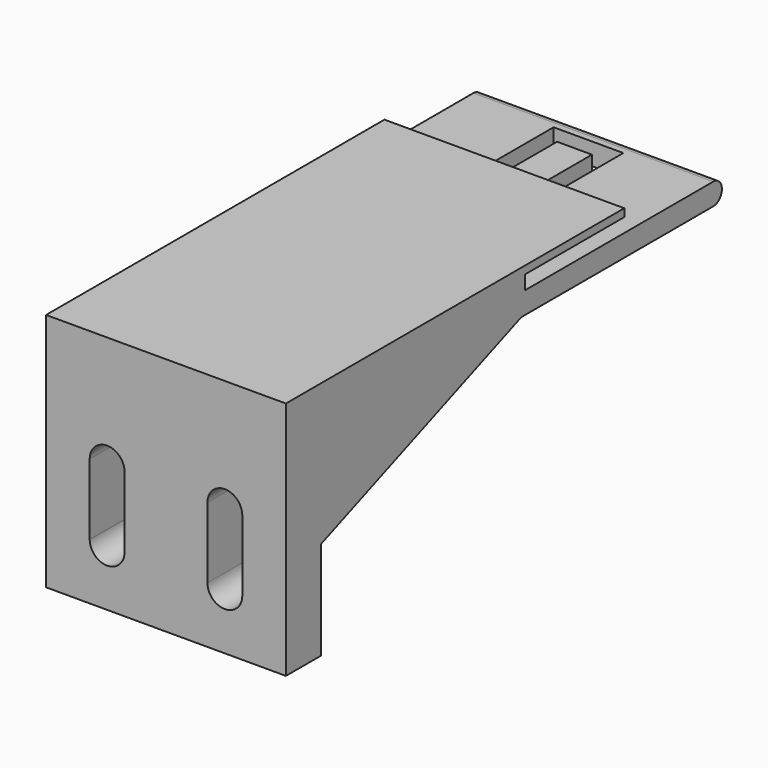
from build123d import *

# Parameters (mm, degrees)
F0_W      = 17.4625
F0_H      = 34.925
F1_DEPTH  = 6.35
F2_W      = 34.925
F2_H      = 6.35
F3_DEPTH  = 73.025
F5_DEPTH  = 3.175
F7_DEPTH  = 3.175
F8_W      = 34.925
F8_H      = 3.175
F9_DEPTH  = 17.78
F10_W     = 34.925
F10_H     = 1.143
F10_H_2   = 0.889
F11_DEPTH = 18.1102
F12_W     = 10.16
F12_H     = 15.24
F13_DEPTH = 25.4
F14_W     = 5.0834602067
F14_H     = 0.7943399184
F14_H_2   = 4.191
F15_DEPTH = 12.7
F17_DEPTH = 5.7404
F18_R     = 1.58749
F19_W     = 5.0834602067
F19_H     = 0.7931600816
F20_DEPTH = 12.7


# Not quite as in the source:
# - a fillet or chamfer is up to 0.001 mm smaller than in the source, because OpenCascade refuses the exact size
# - a feature names something its author has since deleted; it is built from what else it names


with BuildPart() as f1:
    # F0 (on Front) → F1 (new body)
    with BuildSketch(Plane.XZ):
        with Locations((-8.73125, 17.4625)):
            Rectangle(F0_W, F0_H)
        with BuildLine():
            ThreePointArc((-11.43, 18.5185023174), (-8.89, 21.0585023174), (-6.35, 18.5185023174))
            Line((-6.35, 18.5185023174), (-6.35, 8.2149775699))
            ThreePointArc((-6.35, 8.2149775699), (-8.89, 5.6749775699), (-11.43, 8.2149775699))
            Line((-11.43, 8.2149775699), (-11.43, 18.5185023174))
        make_face(mode=Mode.SUBTRACT)
        with Locations((-26.19375, 17.4625)):
            Rectangle(F0_W, F0_H)
        with BuildLine():
            Line((-23.495, 18.5185023174), (-23.495, 8.2149775699))
            ThreePointArc((-23.495, 8.2149775699), (-26.0048819907, 5.6751561381), (-28.5742857524, 8.154745786))
            ThreePointArc((-28.5742857524, 8.154745786), (-28.5748214318, 8.1848595606), (-28.575, 8.2149775699))
            Line((-28.575, 8.2149775699), (-28.575, 18.5185023174))
            ThreePointArc((-28.575, 18.5185023174), (-26.035, 21.0585023174), (-23.495, 18.5185023174))
        make_face(mode=Mode.SUBTRACT)
    extrude(amount=F1_DEPTH)

    # F2 (on face) → F3 (join)
    with BuildSketch(Plane(origin=(0, 0, 0), x_dir=(-1, 0, 0), z_dir=(0, 1, 0))):
        with Locations((17.4625, 31.75)):
            Rectangle(F2_W, F2_H)
    extrude(amount=F3_DEPTH)

    # F4 (on face) → F5 (join)
    with BuildSketch(Plane.YZ):
        Polygon((0, 28.575), (0, 14.2875), (36.5125, 28.575), align=None)
    extrude(amount=-F5_DEPTH)

    # F6 (on face) → F7 (join)
    with BuildSketch(Plane(origin=(-34.925, 0, 0), x_dir=(0, -1, 0), z_dir=(-1, 0, 0))):
        Polygon((-36.5125, 28.575), (0, 14.2875), (0, 28.575), align=None)
    extrude(amount=-F7_DEPTH)

    # F8 (on face) → F9 (cut)
    with BuildSketch(Plane(origin=(0, 73.025, 0), x_dir=(-1, 0, 0), z_dir=(0, 1, 0))):
        with Locations((17.4625, 33.3375)):
            Rectangle(F8_W, F8_H)
    extrude(amount=-F9_DEPTH, mode=Mode.SUBTRACT)

    # F10 (on face) → F11 (cut)
    with BuildSketch(Plane(origin=(0, 55.245, 0), x_dir=(-1, 0, 0), z_dir=(0, 1, 0))):
        with Locations((17.4625, 33.2105)):
            Rectangle(F10_W, F10_H)
        with Locations((17.4625, 32.1945)):
            Rectangle(F10_W, F10_H_2)
    extrude(amount=-F11_DEPTH, mode=Mode.SUBTRACT)

    # F12 (on face) → F13 (cut)
    with BuildSketch(Plane.XY.offset(31.75)):
        with Locations((-17.4625, 62.9390887916)):
            Rectangle(F12_W, F12_H)
    extrude(amount=-F13_DEPTH, mode=Mode.SUBTRACT)

    # F14 (on face) → F15 (join)
    with BuildSketch(Plane(origin=(0, 55.3190887916, 0), x_dir=(-1, 0, 0), z_dir=(0, 1, 0))):
        with Locations((17.4607698967, 30.5596699592)):
            Rectangle(F14_W, F14_H)
        with Locations((17.4607698967, 28.067)):
            Rectangle(F14_W, F14_H_2)
    extrude(amount=F15_DEPTH)

    # F16 (on face) → F17 (cut)
    with BuildSketch(Plane.YZ.offset(-14.9190397933)):
        Polygon((68.0190887916, 28.4641699592), (65.845951438, 25.9715), (67.369951438, 25.9715), (68.0190887916, 25.9715), align=None)
        Polygon((55.3190887916, 25.9715), (62.7900138497, 25.9715), (64.3140138497, 25.9715), (55.3190887916, 29.9881699592), (55.3190887916, 28.575), align=None)
    extrude(amount=-F17_DEPTH, mode=Mode.SUBTRACT)

    # F18 (radius 1.5875 in the source; OpenCascade refuses exactly that, so slightly less here)
    f18_edges = [f1.edges().sort_by_distance(p)[0] for p in [
        (-17.4625, 73.025, 31.75),
        (-17.4625, 73.025, 28.575),
    ]]
    fillet(f18_edges, radius=F18_R)

    # F19 (on face) → F20 (join)
    with BuildSketch(Plane(origin=(0, 55.3190887916, 0), x_dir=(-1, 0, 0), z_dir=(0, 1, 0))):
        with Locations((17.4607698967, 31.3534199592)):
            Rectangle(F19_W, F19_H)
    extrude(amount=F20_DEPTH)


solid = f1.part
